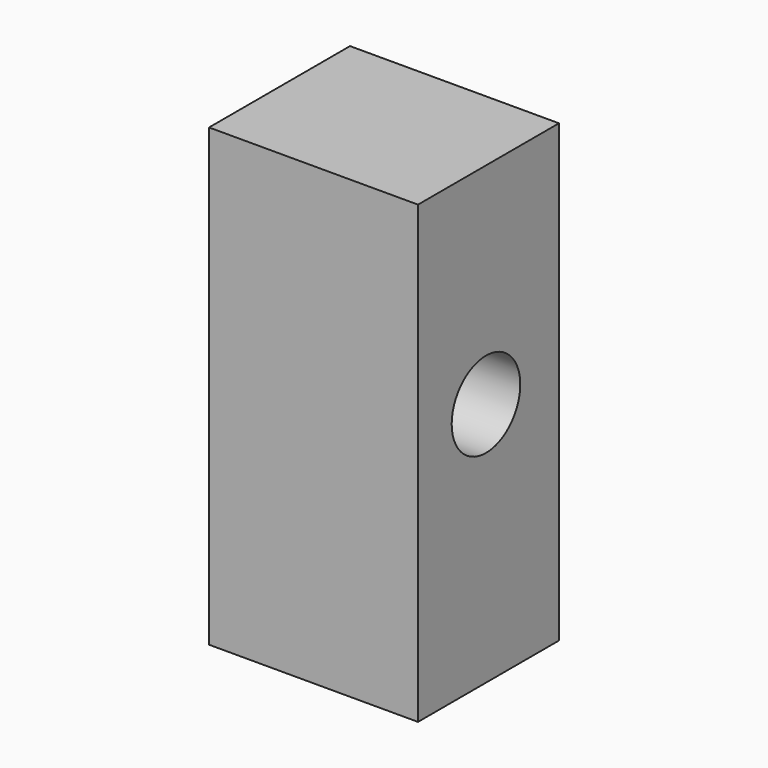
from build123d import *

# Parameters (mm, degrees)
F0_W       = 29.4857565314
F0_H       = 24.8636654578
F1_DEPTH   = 64.262
F2_R       = 6.0488126263
F1_FACE1_W = 24.8636654578
F1_FACE1_H = 64.262
F3_DEPTH   = 36.322


with BuildPart() as f1:
    # F0 (on Top) → F1 (new body)
    with BuildSketch(Plane.XY):
        with Locations((-14.7428782657, 16.4960857946)):
            Rectangle(F0_W, F0_H)
    extrude(amount=F1_DEPTH)

    # F2 (on face) + F1_face1 (on face) → F3 (cut)
    with BuildSketch(Plane(origin=(-29.4857565314, 0, 0), x_dir=(0, -1, 0), z_dir=(-1, 0, 0))):
        with Locations((-16.0558279604, 34.5874093473)):
            Circle(F2_R)
    with BuildSketch(Plane(origin=(0, 16.4960857946, 32.131), x_dir=(0, 1, 0), z_dir=(1, 0, 0))):
        Rectangle(F1_FACE1_W, F1_FACE1_H)
    extrude(amount=-F3_DEPTH, dir=(-1, 0, 0), mode=Mode.SUBTRACT)


solid = f1.part
